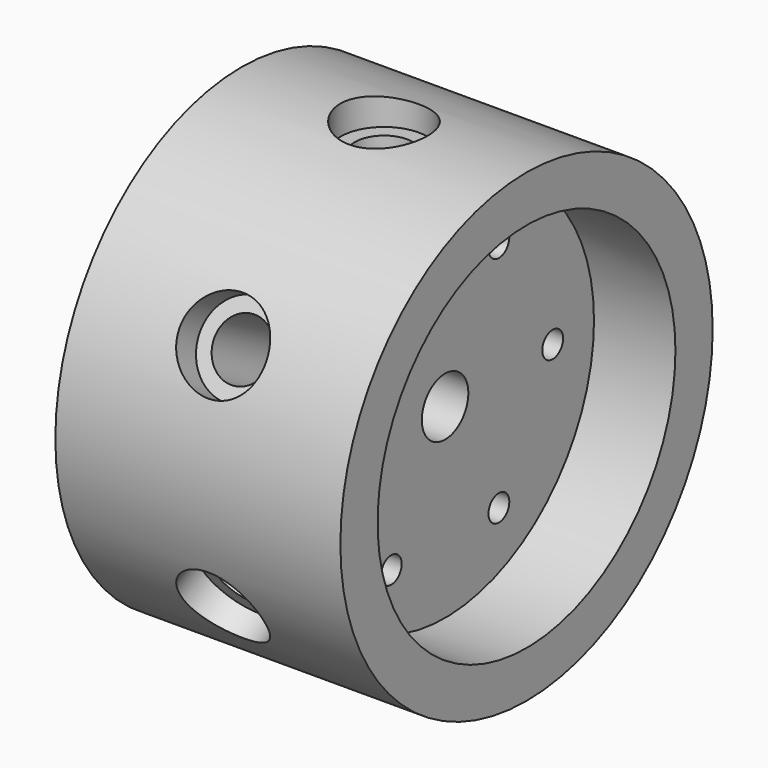
from build123d import *

# Parameters (mm, degrees)
F0_R             = 25.4
F1_DEPTH         = 15.5575
F2_R             = 3.175
F3_DEPTH         = 31.116
F4_R             = 20.32
F5_DEPTH         = 8.89
F6_R             = 1.4224
F7_DEPTH         = 12.7
F9_R             = 4.7625
F9_R_2           = 3.175
F10_DEPTH        = 3.175
F10_COPIES_COUNT = 6
F11_R            = 3.175
F12_DEPTH        = 15.875
F12_COPIES_COUNT = 6


# Not quite as in the source:
# - a pattern or mirror of a feature is missing from the dataset's text; its kind, count and spacing are read off the source's solid


with BuildPart() as f1:
    # F0 (on Right) → F1 (new body, symmetric)
    with BuildSketch(Plane.YZ):
        Circle(F0_R)
    extrude(amount=F1_DEPTH, both=True)

    # F2 (on face) → F3 (cut, through all)
    with BuildSketch(Plane.YZ.offset(15.5575)):
        Circle(F2_R)
    extrude(amount=-F3_DEPTH, mode=Mode.SUBTRACT)

    # F4 (on face) → F5 (cut)
    with BuildSketch(Plane.YZ.offset(15.5575)):
        Circle(F4_R)
    extrude(amount=-F5_DEPTH, mode=Mode.SUBTRACT)

    # F6 (on face) → F7 (cut)
    with BuildSketch(Plane.YZ.offset(6.6675)):
        with Locations((14.6812, 0)):
            Circle(F6_R)
        with Locations((7.3406, -12.714292158)):
            Circle(F6_R)
        with Locations((-7.3406, -12.714292158)):
            Circle(F6_R)
        with Locations((-14.6812, 0)):
            Circle(F6_R)
        with Locations((-7.3406, 12.714292158)):
            Circle(F6_R)
        with Locations((7.3406, 12.714292158)):
            Circle(F6_R)
    extrude(amount=-F7_DEPTH, mode=Mode.SUBTRACT)

    # F9 (on offset) → F10 (cut)
    with BuildSketch(Plane.XY.offset(25.4)):
        Circle(F9_R)
        Circle(F9_R_2, mode=Mode.SUBTRACT)
        Circle(F9_R_2)
    f10 = extrude(amount=-F10_DEPTH, mode=Mode.SUBTRACT)

    # F10_copies: F10 ×6 about axis
    f10_copies_axis = Axis((0, 0, 0), (1, 0, 0))
    for i in range(1, F10_COPIES_COUNT):
        add(f10.rotate(f10_copies_axis, i * 360 / F10_COPIES_COUNT), mode=Mode.SUBTRACT)

    # F11 (on face) → F12 (cut)
    with BuildSketch(Plane.XY.offset(22.225)):
        Circle(F11_R)
    f12 = extrude(amount=-F12_DEPTH, mode=Mode.SUBTRACT)

    # F12_copies: F12 ×6 about axis
    f12_copies_axis = Axis((0, 0, 0), (1, 0, 0))
    for i in range(1, F12_COPIES_COUNT):
        add(f12.rotate(f12_copies_axis, i * 360 / F12_COPIES_COUNT), mode=Mode.SUBTRACT)


solid = f1.part
